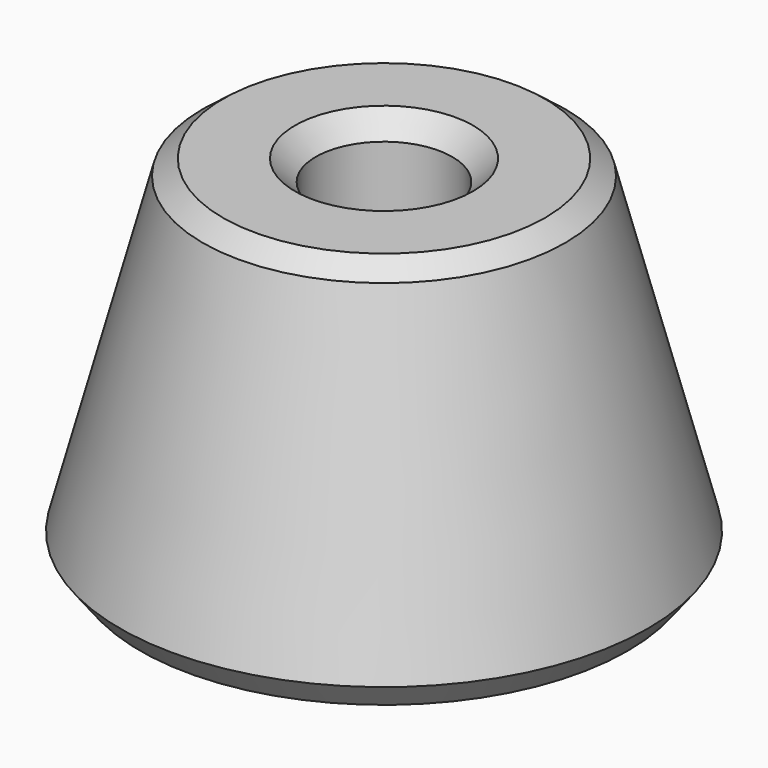
from build123d import *

# Parameters (mm, degrees)
F0_R     = 13
F2_R     = 8.5
F4_R     = 3.275
F5_DEPTH = 25


# Not quite as in the source:
# - a fillet or chamfer that OpenCascade refuses, or shapes differently, is made with other operations: its cross-section is extruded or revolved along the edge and cut away or added


with BuildPart() as f3:
    # F0 (on Top) → F3 section 0
    with BuildSketch(Plane.XY):
        Circle(F0_R)
    # F2 (on offset) → F3 section 1
    with BuildSketch(Plane.XY.offset(17)):
        Circle(F2_R)
    loft()

    # F4 (on face) → F5 (cut)
    with BuildSketch(Plane.XY.offset(17)):
        Circle(F4_R)
    extrude(amount=-F5_DEPTH, mode=Mode.SUBTRACT)

    # F6: chamfer of 1 on 4 edges, made by hand

    # F6_s1 → F6_t2 (revolve, cut)
    with BuildSketch(Plane.XZ):
        Polygon((4.275, 17), (3.275, 16), (3.275, 17), align=None)
    revolve(axis=Axis((0, 0, 17), (0, 0, 1)), mode=Mode.SUBTRACT)

    # F6_s3 → F6_t4 (revolve, cut)
    with BuildSketch(Plane.XZ):
        Polygon((8.6969696164, 16.2558925603), (7.7302643885, 17), (8.5, 17), align=None)
    revolve(axis=Axis((0, 0, 17), (0, 0, 1)), mode=Mode.SUBTRACT)

    # F6_s5 → F6_t6 (revolve, cut)
    with BuildSketch(Plane.XZ):
        Polygon((12.6675578517, 1.2558925603), (11.7008526238, 0), (13, 0), align=None)
    revolve(axis=Axis((0, 0, 0), (0, 0, 1)), mode=Mode.SUBTRACT)

    # F6_s7 → F6_t8 (revolve, cut)
    with BuildSketch(Plane.XZ):
        Polygon((4.275, 0), (3.275, 1), (3.275, 0), align=None)
    revolve(axis=Axis((0, 0, 0), (0, 0, 1)), mode=Mode.SUBTRACT)


solid = f3.part
